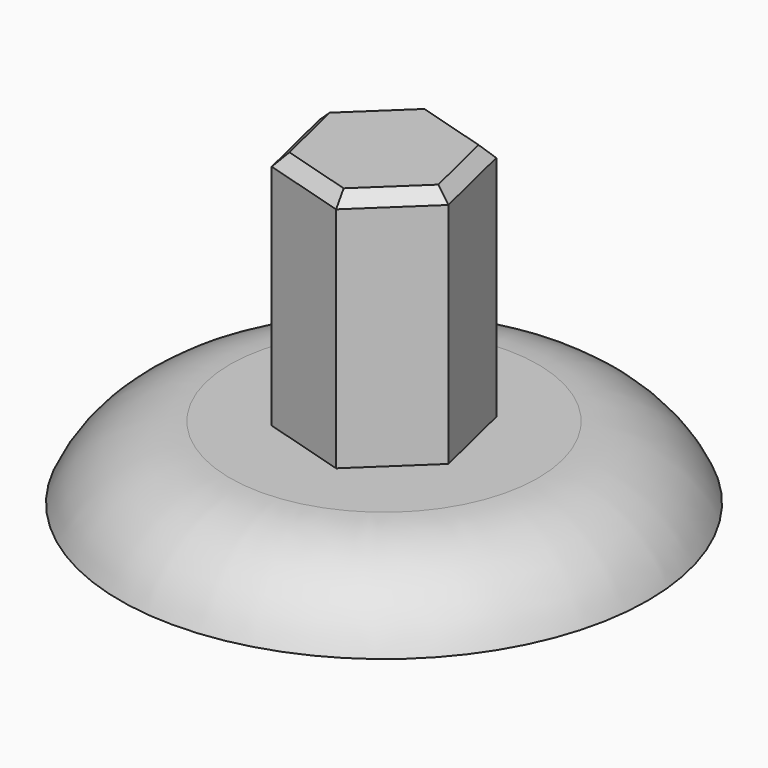
from build123d import *

# Parameters (mm, degrees)
F0_R     = 11
F1_DEPTH = 3
F3_DEPTH = 10
F4_SIZE  = 0.5


# Not quite as in the source:
# - a fillet or chamfer that OpenCascade refuses, or shapes differently, is made with other operations: its cross-section is extruded or revolved along the edge and cut away or added


with BuildPart() as f1:
    # F0 (on Top) → F1 (new body)
    with BuildSketch(Plane.XY):
        Circle(F0_R)
    extrude(amount=F1_DEPTH)

    # F2 (on face) → F3 (join)
    with BuildSketch(Plane.XY.offset(3)):
        Polygon((0.8564302523, -3.5647384976), (3.5153692229, -1.0406788937), (2.6589389706, 2.5240596039), (-0.8564302523, 3.5647384976), (-3.5153692229, 1.0406788937), (-2.6589389706, -2.5240596039), align=None)
    extrude(amount=F3_DEPTH)

    # F4
    f4_edges = [f1.edges().sort_by_distance(p)[0] for p in [
        (2.1859, -2.302709, 13),
        (3.087154, 0.74169, 13),
        (0.901254, 3.044399, 13),
        (-2.1859, 2.302709, 13),
        (-3.087154, -0.74169, 13),
        (-0.901254, -3.044399, 13),
    ]]
    chamfer(f4_edges, length=F4_SIZE)

    # F5: fillet of radius 5 on 1 edges, made by hand

    # F5_s1 → F5_t2 (revolve, cut)
    with BuildSketch(Plane.XZ):
        with BuildLine():
            ThreePointArc((6.417424305, 3), (9.1560370926, 2.1833001327), (11, 0))
            Line((11, 0), (11, 3))
            Line((11, 3), (6.417424305, 3))
        make_face()
    revolve(axis=Axis((0, 0, 3), (0, 0, 1)), mode=Mode.SUBTRACT)


solid = f1.part
